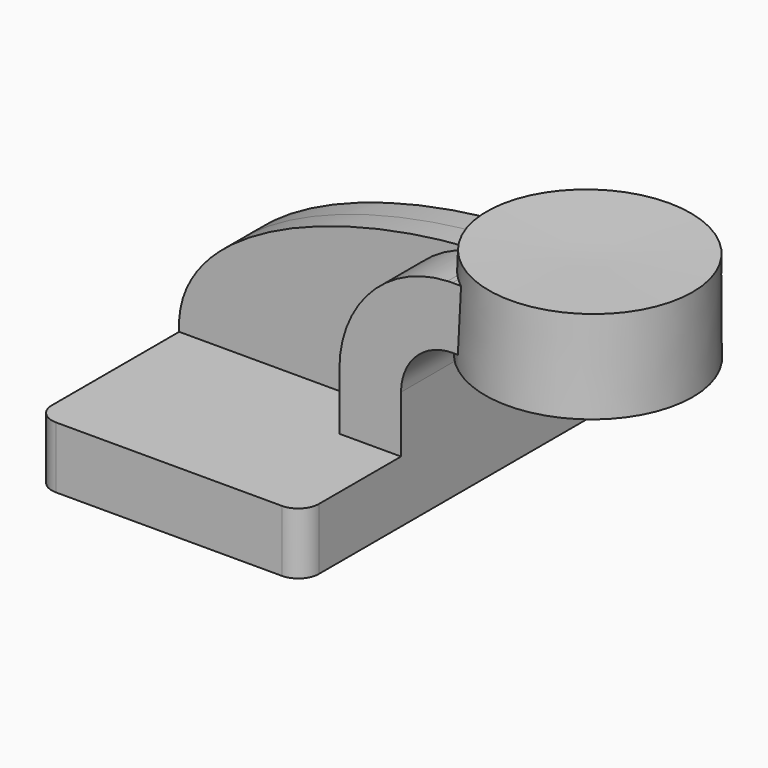
from build123d import *

# Parameters (mm, degrees)
F1_DEPTH = 63.5
F2_DEPTH = 25.4
F3_DEPTH = 7.9375
F4_DEPTH = 25.4
F6_R     = 6.35


# Not quite as in the source:
# - a feature names something its author has since deleted; it is built from what else it names


with BuildPart() as f1:
    # F0 (on Front) → F1 (new body, symmetric)
    with BuildSketch(Plane.XZ):
        Polygon((22.225, 9.525), (-41.275, 9.525), (-41.275, -9.525), (41.275, -9.525), (41.275, 9.525), align=None)
    extrude(amount=F1_DEPTH, both=True)

    # F0 (on Front) → F2 (join, symmetric)
    with BuildSketch(Plane.XZ):
        with BuildLine():
            Line((22.225, 27.051), (22.225, 9.525))
            Line((22.225, 9.525), (41.275, 9.525))
            Line((41.275, 9.525), (41.275, 27.051))
            ThreePointArc((41.275, 27.051), (45.9246798487, 38.2763201513), (57.15, 42.926))
            Line((57.15, 42.926), (60.325, 42.926))
            Line((60.325, 42.926), (60.325, 61.976))
            Line((60.325, 61.976), (57.15, 61.976))
            add(Edge.make_bspline(
                [(55.6844107211, 61.9452355277), (56.1739766533, 61.9576548863), (56.6625337097, 61.9679123237), (57.15, 61.976)],
                knots=[110.3317061333, 110.3317061333, 110.3317061333, 110.3317061333, 111.5284180198, 111.5284180198, 111.5284180198, 111.5284180198], degree=3))
            ThreePointArc((55.6844107211, 61.9452355277), (31.9414565021, 51.2229870866), (22.225, 27.051))
        make_face()
    extrude(amount=F2_DEPTH, both=True)

    # F0 (on Front) → F3 (join, symmetric)
    with BuildSketch(Plane.XZ):
        with BuildLine():
            add(Edge.make_bspline(
                [(-41.275, 9.525), (-43.1628450735, 41.2787763348), (10.5485303307, 60.8002239091), (55.6844107211, 61.9452355277)],
                knots=[0, 0, 0, 0, 110.3317061333, 110.3317061333, 110.3317061333, 110.3317061333], degree=3))
            Line((-41.275, 9.525), (22.225, 9.525))
            Line((22.225, 9.525), (22.225, 27.051))
            ThreePointArc((22.225, 27.051), (31.9414565021, 51.2229870866), (55.6844107211, 61.9452355277))
        make_face()
    extrude(amount=F3_DEPTH, both=True)

    # F0 (on Front) → F4 (join, symmetric)
    with BuildSketch(Plane.XZ):
        Polygon((79.1998635302, 61.976), (60.325, 61.976), (60.325, 42.926), (78.823101495, 42.926), align=None)
    extrude(amount=F4_DEPTH, both=True)

    # F0 (on Front) → F5 (revolve)
    with BuildSketch(Plane.XZ):
        Polygon((79.2927981655, 66.675), (79.1998635302, 61.976), (78.823101495, 42.926), (78.7276551127, 38.1), (111.125, 38.1), (111.125, 66.675), align=None)
    revolve(axis=Axis((79.0102266391, 0, 52.3875), (0.0197736678, 0, 0.9998044819)))

    # F6
    f6_edges = [f1.edges().sort_by_distance(p)[0] for p in [
        (41.275, -63.5, 0),
        (-41.275, -63.5, 0),
        (-41.275, 63.5, 0),
        (41.275, 63.5, 0),
    ]]
    fillet(f6_edges, radius=F6_R)


solid = f1.part
